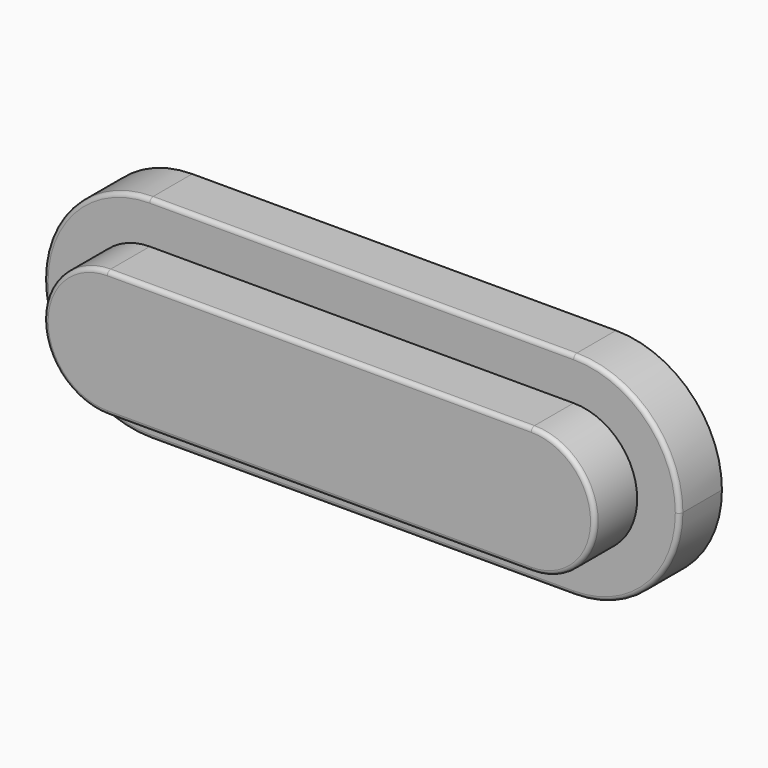
from build123d import *

# Parameters (mm, degrees)
F1_DEPTH = 50
F2_DEPTH = 25
F3_R     = 2


with BuildPart() as f1:
    # F0 (on Front) → F1 (new body)
    with BuildSketch(Plane.XZ):
        with BuildLine():
            Line((-100, -30), (100, -30))
            ThreePointArc((100, -30), (121.2132034356, -21.2132034356), (130, 0))
            ThreePointArc((130, 0), (121.2132034356, 21.2132034356), (100, 30))
            Line((100, 30), (-100, 30))
            ThreePointArc((-100, 30), (-121.2132034356, 21.2132034356), (-130, 0))
            ThreePointArc((-130, 0), (-121.2132034356, -21.2132034356), (-100, -30))
        make_face()
    extrude(amount=F1_DEPTH)

    # F0 (on Front) → F2 (join)
    with BuildSketch(Plane.XZ):
        with BuildLine():
            Line((-100, -50), (100, -50))
            ThreePointArc((100, -50), (135.3553390593, -35.3553390593), (150, 0))
            ThreePointArc((150, 0), (135.3553390593, 35.3553390593), (100, 50))
            Line((100, 50), (-100, 50))
            ThreePointArc((-100, 50), (-135.3553390593, 35.3553390593), (-150, 0))
            ThreePointArc((-150, 0), (-135.3553390593, -35.3553390593), (-100, -50))
        make_face()
        with BuildLine():
            ThreePointArc((130, 0), (121.2132034356, -21.2132034356), (100, -30))
            Line((100, -30), (-100, -30))
            ThreePointArc((-100, -30), (-121.2132034356, -21.2132034356), (-130, 0))
            ThreePointArc((-130, 0), (-121.2132034356, 21.2132034356), (-100, 30))
            Line((-100, 30), (100, 30))
            ThreePointArc((100, 30), (121.2132034356, 21.2132034356), (130, 0))
        make_face(mode=Mode.SUBTRACT)
    extrude(amount=F2_DEPTH)

    # F3
    f3_edges = [f1.edges().sort_by_distance(p)[0] for p in [
        (-150, -25, 0),
        (0, -50, -30),
        (0, -25, -50),
        (150, -25, 0),
        (0, -25, 50),
        (130, -50, 0),
        (0, -50, 30),
        (-130, -50, 0),
    ]]
    fillet(f3_edges, radius=F3_R)


solid = f1.part
